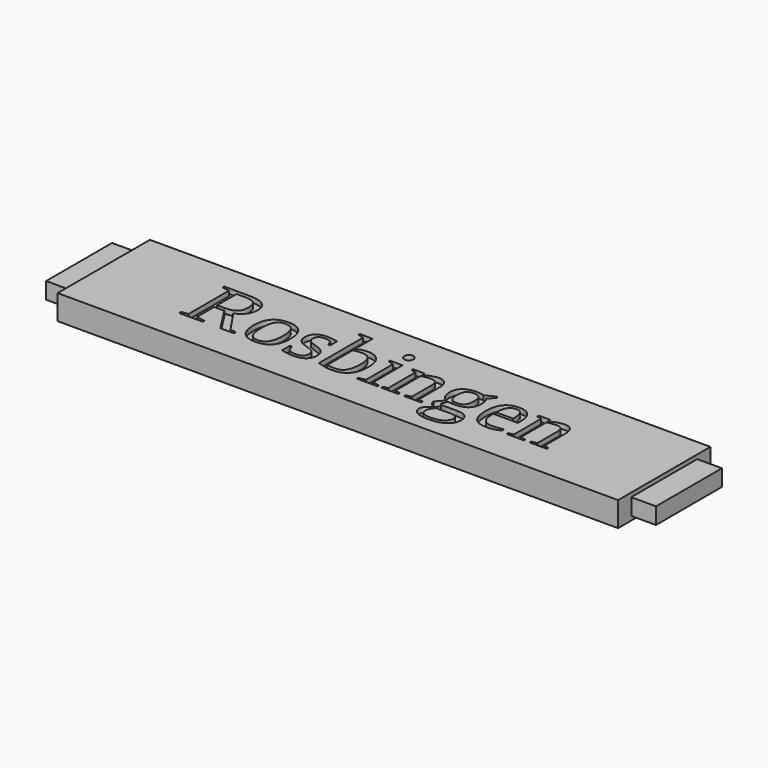
from build123d import *

# Parameters (mm, degrees)
F0_W         = 340
F0_H         = 70
F1_DEPTH     = 15
F2_W         = 50
F2_H         = 10
F3_DEPTH     = 15
F4_W         = 50
F4_H         = 10
F5_DEPTH     = 15
F6_TEXT_SIZE = 52.7777777778
F7_DEPTH     = 3


# Not quite as in the source:
# - Text() gives the source's letters only with a copy of the font that has no kerning and outlines rounded to 1/6400 em; it was checked with that copy


with BuildPart() as f1:
    # F0 (on Top) → F1 (new body)
    with BuildSketch(Plane.XY):
        with Locations((1.1496338993, 45.7458090895)):
            Rectangle(F0_W, F0_H)
    extrude(amount=F1_DEPTH)

    # F2 (on face) → F3 (join)
    with BuildSketch(Plane.YZ.offset(171.1496338993)):
        with Locations((45.7458090895, 7.5)):
            Rectangle(F2_W, F2_H)
    extrude(amount=F3_DEPTH)

    # F4 (on face) → F5 (join)
    with BuildSketch(Plane(origin=(-168.8503661007, 0, 0), x_dir=(0, -1, 0), z_dir=(-1, 0, 0))):
        with Locations((-45.7458090895, 7.5)):
            Rectangle(F4_W, F4_H)
    extrude(amount=F5_DEPTH)

    # F6 (on face) → F7 (cut)
    with BuildSketch(Plane.XY.offset(15)):
        with Locations((-112.9905570729, 30.7458090895)):
            Text('Rosbingen', F6_TEXT_SIZE, font='Tinos', text_align=(TextAlign.LEFT, TextAlign.BOTTOM))
    extrude(amount=-F7_DEPTH, mode=Mode.SUBTRACT)


solid = f1.part
